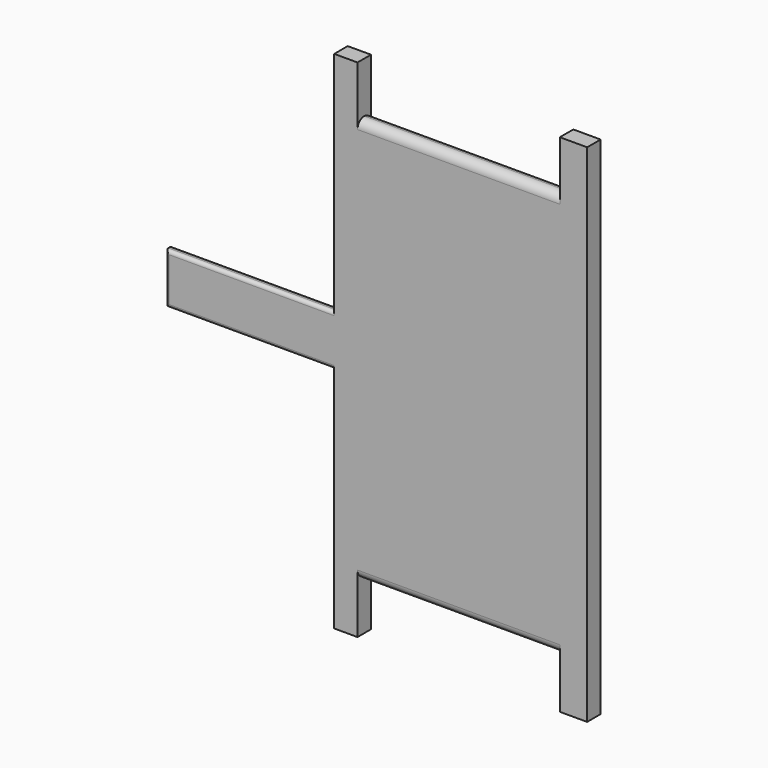
from build123d import *

# Parameters (mm, degrees)
F0_W     = 10
F0_H     = 3
F1_DEPTH = 1
F2_DEPTH = 0.5
F3_R     = 0.2
F4_R     = 0.49999


# Not quite as in the source:
# - a fillet or chamfer is up to 0.001 mm smaller than in the source, because OpenCascade refuses the exact size


with BuildPart() as f1:
    # F0 (on Front) → F1 (new body)
    with BuildSketch(Plane.XZ):
        with Locations((-12.5, 0.0299999826)):
            Rectangle(F0_W, F0_H)
        Polygon((-6.1200000346, 15), (-7.5, 15), (-7.5, 1.5299999826), (-7.5, -1.4700000174), (-7.5, -15), (-6.1200000346, -15), (-6.1200000346, -12), (5.8799999654, -12), (5.8799999654, -15), (7.5, -15), (7.5, 15), (5.8799999654, 15), (5.8799999654, 12), (-6.1200000346, 12), align=None)
    extrude(amount=F1_DEPTH)

    # F0 (on Front) → F2 (cut)
    with BuildSketch(Plane.XZ):
        with Locations((-12.5, 0.0299999826)):
            Rectangle(F0_W, F0_H)
    extrude(amount=F2_DEPTH, mode=Mode.SUBTRACT)

    # F3
    f3_edges = [f1.edges().sort_by_distance(p)[0] for p in [
        (-12.5, -0.5, -1.47),
        (-12.5, -0.5, 1.53),
        (-12.5, -1, -1.47),
        (-12.5, -1, 1.53),
        (-17.5, -1, 0.03),
        (-17.5, -0.5, 0.03),
    ]]
    fillet(f3_edges, radius=F3_R)

    # F4 (radius 0.5 in the source; OpenCascade refuses exactly that, so slightly less here)
    f4_edges = [f1.edges().sort_by_distance(p)[0] for p in [
        (-0.12, -1, -12),
        (-0.12, -1, 12),
        (-0.12, 0, -12),
        (-0.12, 0, 12),
    ]]
    fillet(f4_edges, radius=F4_R)


solid = f1.part
